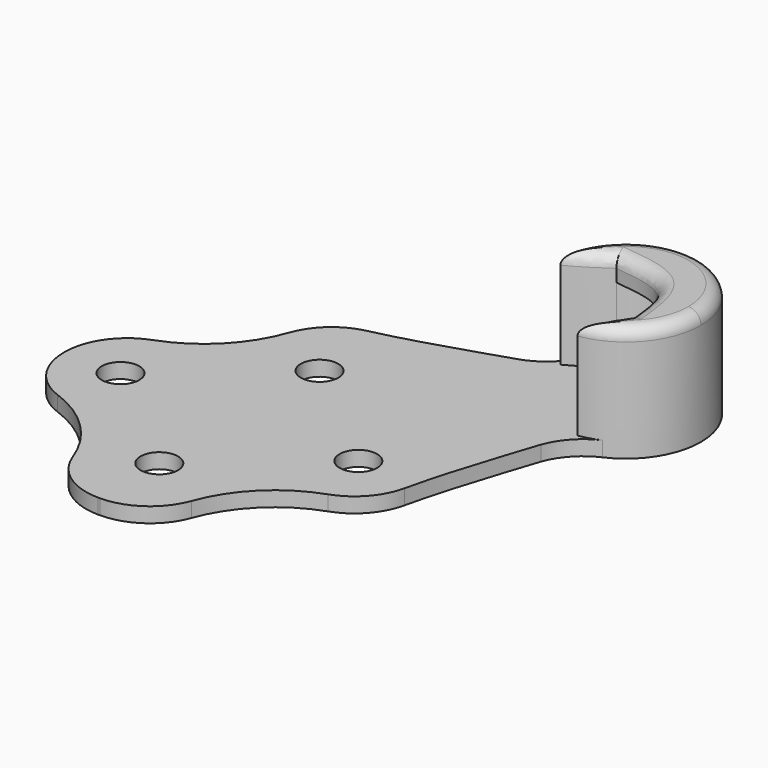
from build123d import *

# Parameters (mm, degrees)
F0_R     = 3
F0_R_2   = 1.5
F1_DEPTH = 1.2
F2_R     = 5
F3_DEPTH = 9.2
F4_START = 1.2
F4_DEPTH = 6
F5_R     = 1


# Not quite as in the source:
# - a feature names something its author has since deleted; it is built from what else it names


with BuildPart() as f1:
    # F0 (on Top) → F1 (new body)
    with BuildSketch(Plane.XY):
        with BuildLine():
            ThreePointArc((-4.1724739695, 13.3637742039), (-7.0710678119, 7.0710678119), (-13.3637742039, 4.1724739695))
            ThreePointArc((-13.3637742039, 4.1724739695), (-14, 0), (-13.3637742039, -4.1724739695))
            ThreePointArc((-13.3637742039, -4.1724739695), (-7.0710678119, -7.0710678119), (-4.1724739695, -13.3637742039))
            ThreePointArc((-4.1724739695, -13.3637742039), (0, -14), (4.1724739695, -13.3637742039))
            ThreePointArc((4.1724739695, -13.3637742039), (7.0710678119, -7.0710678119), (13.3637742039, -4.1724739695))
            ThreePointArc((13.3637742039, -4.1724739695), (13.6514806081, -3.1043642196), (13.8539604417, -2.0168738382))
            add(Edge.make_bspline(
                [(18.0302855152, 11.2126611682), (17.2036823376, 9.5946472755), (16.1235417051, 6.0326561447), (14.4969162211, 1.1586980327), (13.8539604417, -2.0168738382)],
                knots=[0.1747836978, 0.1747836978, 0.1747836978, 0.1747836978, 0.4899837787, 1, 1, 1, 1], degree=3))
            ThreePointArc((18.0302855152, 11.2126611682), (12.9046987567, 12.9046987567), (11.2126611682, 18.0302855152))
            add(Edge.make_bspline(
                [(11.2126611682, 18.0302855152), (9.5946472755, 17.2036823376), (6.0326561447, 16.1235417051), (1.1586980327, 14.4969162211), (-2.0168738382, 13.8539604417)],
                knots=[0.1747836978, 0.1747836978, 0.1747836978, 0.1747836978, 0.4899837787, 1, 1, 1, 1], degree=3))
            ThreePointArc((-2.0168738382, 13.8539604417), (-3.1043642196, 13.6514806081), (-4.1724739695, 13.3637742039))
        make_face()
        with Locations((0, -8)):
            Circle(F0_R, mode=Mode.SUBTRACT)
        with Locations((-9.5, 0)):
            Circle(F0_R, mode=Mode.SUBTRACT)
        with Locations((9.5, 0)):
            Circle(F0_R, mode=Mode.SUBTRACT)
        with Locations((0, 8)):
            Circle(F0_R, mode=Mode.SUBTRACT)
        with BuildLine():
            add(Edge.make_bspline(
                [(14.2183567736, 19.8715017954), (13.0862627872, 19.074326183), (12.1098768368, 18.4886507529), (11.2126611682, 18.0302855152)],
                knots=[0, 0, 0, 0, 0.1747836978, 0.1747836978, 0.1747836978, 0.1747836978], degree=3))
            ThreePointArc((11.2126611682, 18.0302855152), (12.9046987567, 12.9046987567), (18.0302855152, 11.2126611682))
            add(Edge.make_bspline(
                [(19.8715017954, 14.2183567736), (19.074326183, 13.0862627872), (18.4886507529, 12.1098768368), (18.0302855152, 11.2126611682)],
                knots=[0, 0, 0, 0, 0.1747836978, 0.1747836978, 0.1747836978, 0.1747836978], degree=3))
            ThreePointArc((19.8715017954, 14.2183567736), (14.318912319, 14.318912319), (14.2183567736, 19.8715017954))
        make_face()
        with BuildLine():
            ThreePointArc((23.1473394438, 17.1473394438), (17.5900189816, 23.1309867284), (11.2126611682, 18.0302855152))
            add(Edge.make_bspline(
                [(14.2183567736, 19.8715017954), (13.0862627872, 19.074326183), (12.1098768368, 18.4886507529), (11.2126611682, 18.0302855152)],
                knots=[0, 0, 0, 0, 0.1747836978, 0.1747836978, 0.1747836978, 0.1747836978], degree=3))
            ThreePointArc((14.2183567736, 19.8715017954), (18.6109085948, 20.869968265), (21.1473394438, 17.1473394438))
            ThreePointArc((21.1473394438, 17.1473394438), (20.8145351985, 15.5499430319), (19.8715017954, 14.2183567736))
            add(Edge.make_bspline(
                [(19.8715017954, 14.2183567736), (19.074326183, 13.0862627872), (18.4886507529, 12.1098768368), (18.0302855152, 11.2126611682)],
                knots=[0, 0, 0, 0, 0.1747836978, 0.1747836978, 0.1747836978, 0.1747836978], degree=3))
            ThreePointArc((18.0302855152, 11.2126611682), (21.691438718, 13.2292835756), (23.1473394438, 17.1473394438))
        make_face()
        with BuildLine():
            add(Edge.make_bspline(
                [(14.2183567736, 19.8715017954), (15.9188594714, 19.6876228193), (19.319864867, 19.319864867), (19.6876228193, 15.9188594714), (19.8715017954, 14.2183567736)],
                knots=[0, 0, 0, 0, 0.5, 1, 1, 1, 1], degree=3))
            ThreePointArc((14.2183567736, 19.8715017954), (14.318912319, 14.318912319), (19.8715017954, 14.2183567736))
        make_face()
        with Locations((9.5, 0)):
            Circle(F0_R)
        with Locations((9.5, 0)):
            Circle(F0_R_2, mode=Mode.SUBTRACT)
        with Locations((0, 8)):
            Circle(F0_R)
        with Locations((0, 8)):
            Circle(F0_R_2, mode=Mode.SUBTRACT)
        with Locations((-9.5, 0)):
            Circle(F0_R)
        with Locations((-9.5, 0)):
            Circle(F0_R_2, mode=Mode.SUBTRACT)
        with Locations((0, -8)):
            Circle(F0_R)
        with Locations((0, -8)):
            Circle(F0_R_2, mode=Mode.SUBTRACT)
        with BuildLine():
            ThreePointArc((21.1473394438, 17.1473394438), (18.6109085948, 20.869968265), (14.2183567736, 19.8715017954))
            add(Edge.make_bspline(
                [(14.2183567736, 19.8715017954), (15.9188594714, 19.6876228193), (19.319864867, 19.319864867), (19.6876228193, 15.9188594714), (19.8715017954, 14.2183567736)],
                knots=[0, 0, 0, 0, 0.5, 1, 1, 1, 1], degree=3))
            ThreePointArc((19.8715017954, 14.2183567736), (20.8145351985, 15.5499430319), (21.1473394438, 17.1473394438))
        make_face()
    extrude(amount=F1_DEPTH)

    # F2
    f2_edges = [f1.edges().sort_by_distance(p)[0] for p in [
        (11.212661, 18.030286, 0.6),
        (18.030286, 11.212661, 0.6),
        (-4.172474, 13.363774, 0.6),
        (-13.363774, 4.172474, 0.6),
        (-13.363774, -4.172474, 0.6),
        (-4.172474, -13.363774, 0.6),
        (4.172474, -13.363774, 0.6),
        (13.363774, -4.172474, 0.6),
    ]]
    fillet(f2_edges, radius=F2_R)

    # F0 (on Top) → F3 (join)
    with BuildSketch(Plane.XY):
        with BuildLine():
            ThreePointArc((23.1473394438, 17.1473394438), (17.5900189816, 23.1309867284), (11.2126611682, 18.0302855152))
            add(Edge.make_bspline(
                [(14.2183567736, 19.8715017954), (13.0862627872, 19.074326183), (12.1098768368, 18.4886507529), (11.2126611682, 18.0302855152)],
                knots=[0, 0, 0, 0, 0.1747836978, 0.1747836978, 0.1747836978, 0.1747836978], degree=3))
            ThreePointArc((14.2183567736, 19.8715017954), (18.6109085948, 20.869968265), (21.1473394438, 17.1473394438))
            ThreePointArc((21.1473394438, 17.1473394438), (20.8145351985, 15.5499430319), (19.8715017954, 14.2183567736))
            add(Edge.make_bspline(
                [(19.8715017954, 14.2183567736), (19.074326183, 13.0862627872), (18.4886507529, 12.1098768368), (18.0302855152, 11.2126611682)],
                knots=[0, 0, 0, 0, 0.1747836978, 0.1747836978, 0.1747836978, 0.1747836978], degree=3))
            ThreePointArc((18.0302855152, 11.2126611682), (21.691438718, 13.2292835756), (23.1473394438, 17.1473394438))
        make_face()
        with BuildLine():
            ThreePointArc((21.1473394438, 17.1473394438), (18.6109085948, 20.869968265), (14.2183567736, 19.8715017954))
            add(Edge.make_bspline(
                [(14.2183567736, 19.8715017954), (15.9188594714, 19.6876228193), (19.319864867, 19.319864867), (19.6876228193, 15.9188594714), (19.8715017954, 14.2183567736)],
                knots=[0, 0, 0, 0, 0.5, 1, 1, 1, 1], degree=3))
            ThreePointArc((19.8715017954, 14.2183567736), (20.8145351985, 15.5499430319), (21.1473394438, 17.1473394438))
        make_face()
    extrude(amount=F3_DEPTH)

    # F0 (on Top) → F4 (cut)
    with BuildSketch(Plane.XY.offset(F4_START)):
        with BuildLine():
            ThreePointArc((21.1473394438, 17.1473394438), (18.6109085948, 20.869968265), (14.2183567736, 19.8715017954))
            add(Edge.make_bspline(
                [(14.2183567736, 19.8715017954), (15.9188594714, 19.6876228193), (19.319864867, 19.319864867), (19.6876228193, 15.9188594714), (19.8715017954, 14.2183567736)],
                knots=[0, 0, 0, 0, 0.5, 1, 1, 1, 1], degree=3))
            ThreePointArc((19.8715017954, 14.2183567736), (20.8145351985, 15.5499430319), (21.1473394438, 17.1473394438))
        make_face()
    extrude(amount=F4_DEPTH, mode=Mode.SUBTRACT)

    # F5
    f5_edges = [f1.edges().sort_by_distance(p)[0] for p in [
        (21.38998, 21.38998, 9.2),
        (18.561553, 18.561553, 9.2),
        (18.897757, 12.747934, 9.2),
        (12.747934, 18.897757, 9.2),
    ]]
    fillet(f5_edges, radius=F5_R)


solid = f1.part
